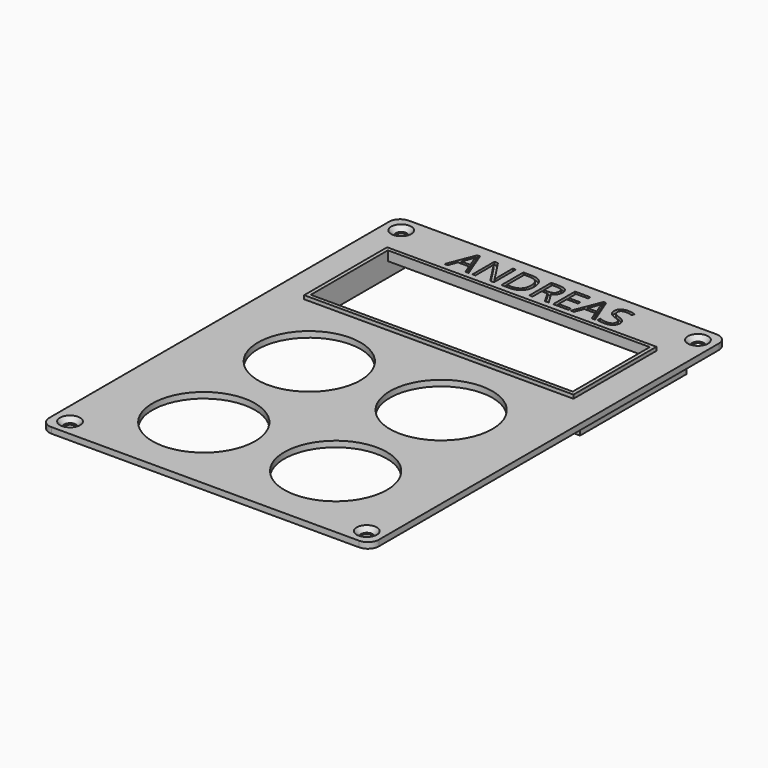
from build123d import *

# Parameters (mm, degrees)
F0_R           = 1.55
F0_R_2         = 14
F0_W           = 71.5
F0_H           = 26.3
F1_DEPTH       = 1.6
F2_TEXT_SIZE   = 10.4795290756
F3_DEPTH       = 0.8
F4_W           = 73.4999993473
F4_H           = 28.2999993473
F4_W_2         = 71.5
F4_H_2         = 26.3
F5_DEPTH       = 1
F7_DEPTH       = 4
F9_D           = 3.1
F9_CSINK_D     = 5.5
F9_CSINK_ANGLE = 90


# Not quite as in the source:
# - a feature names something its author has since deleted; it is built from what else it names
# - Text() gives the source's letters only with a copy of the font that has no kerning and outlines rounded to 1/6400 em; it was checked with that copy


with BuildPart() as f1:
    # F0 (on Top) → F1 (new body)
    with BuildSketch(Plane.XY):
        with BuildLine():
            Line((-42, -93.85), (42, -93.85))
            ThreePointArc((42, -93.85), (44.1213203436, -92.9713203436), (45, -90.85))
            Line((45, -90.85), (45, 25.15))
            ThreePointArc((45, 25.15), (44.1213203436, 27.2713203436), (42, 28.15))
            Line((42, 28.15), (-42, 28.15))
            ThreePointArc((-42, 28.15), (-44.1213203436, 27.2713203436), (-45, 25.15))
            Line((-45, 25.15), (-45, -90.85))
            ThreePointArc((-45, -90.85), (-44.1213203436, -92.9713203436), (-42, -93.85))
        make_face()
        with Locations((-40.5, -89.35)):
            Circle(F0_R, mode=Mode.SUBTRACT)
        with Locations((-18, -71.85)):
            Circle(F0_R_2, mode=Mode.SUBTRACT)
        with Locations((-18, -35.85)):
            Circle(F0_R_2, mode=Mode.SUBTRACT)
        with Locations((18, -71.85)):
            Circle(F0_R_2, mode=Mode.SUBTRACT)
        with Locations((40.5, -89.35)):
            Circle(F0_R, mode=Mode.SUBTRACT)
        with Locations((18, -35.85)):
            Circle(F0_R_2, mode=Mode.SUBTRACT)
        with Locations((-40.5, 23.65)):
            Circle(F0_R, mode=Mode.SUBTRACT)
        Rectangle(F0_W, F0_H, mode=Mode.SUBTRACT)
        with Locations((40.5, 23.65)):
            Circle(F0_R, mode=Mode.SUBTRACT)
    extrude(amount=F1_DEPTH)

    # F2 (on face) → F3 (cut)
    with BuildSketch(Plane.XY.offset(1.6)):
        with Locations((-23.5863402288, 17.2451193686)):
            Text('ANDREAS', F2_TEXT_SIZE, font='Open Sans', text_align=(TextAlign.LEFT, TextAlign.BOTTOM))
    extrude(amount=-F3_DEPTH, mode=Mode.SUBTRACT)

    # F4 (on face) → F5 (join)
    with BuildSketch(Plane.XY.offset(1.6)):
        Rectangle(F4_W, F4_H)
        Rectangle(F4_W_2, F4_H_2, mode=Mode.SUBTRACT)
    extrude(amount=F5_DEPTH)

    # F6 (on face) → F7 (join)
    with BuildSketch(Plane(origin=(0, 0, 0), x_dir=(1, 0, 0), z_dir=(0, 0, -1))):
        Polygon((35.75, -18.15), (41.75, -18.15), (41.75, 18.15), (35.75, 18.15), (35.75, 13.15), (35.75, -13.15), align=None)
        Polygon((-35.75, -18.8523735851), (-35.75, -13.15), (-35.75, 13.15), (-35.75, 17.4476264149), (-41.75, 17.4476264149), (-41.75, -18.8523735851), align=None)
    extrude(amount=F7_DEPTH)

    # F9 (through all)
    with Locations(Plane.XY.offset(1.6)):
        with Locations((-40.5, 23.65), (40.5, 23.65), (-40.5, -89.35), (40.5, -89.35)):
            CounterSinkHole(F9_D / 2, F9_CSINK_D / 2, counter_sink_angle=F9_CSINK_ANGLE)


solid = f1.part
